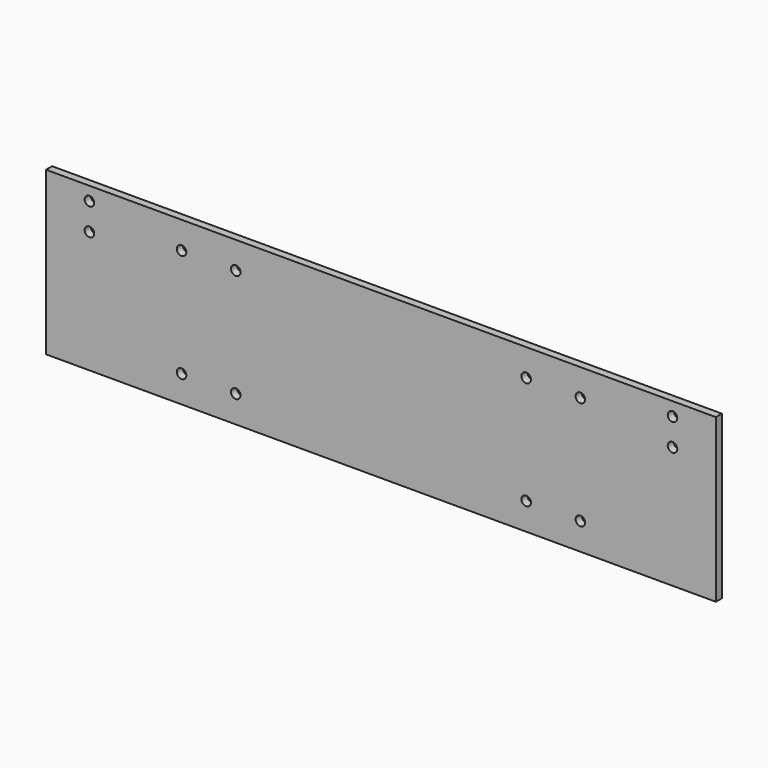
from build123d import *

# Parameters (mm, degrees)
F0_W     = 618
F0_H     = 150
F1_DEPTH = 7
F3_D     = 8.8
F5_D     = 8.8


# Not quite as in the source:
# - a feature names something its author has since deleted; it is built from what else it names


with BuildPart() as f1:
    # F0 (on Front) → F1 (new body)
    with BuildSketch(Plane.XZ):
        with Locations((1, -375)):
            Rectangle(F0_W, F0_H)
    extrude(amount=F1_DEPTH)

    # F3 (through all)
    with Locations(Plane.XZ.offset(7)):
        with Locations((-183, -325), (-133, -325), (185, -325), (185, -425), (135, -425), (-133, -425), (-183, -425), (135, -325)):
            Hole(F3_D / 2)

    # F5 (through all)
    with Locations(Plane.XZ.offset(7)):
        with Locations((-268, -337.5), (-268, -312.5), (270, -337.5), (270, -312.5)):
            Hole(F5_D / 2)


solid = f1.part
